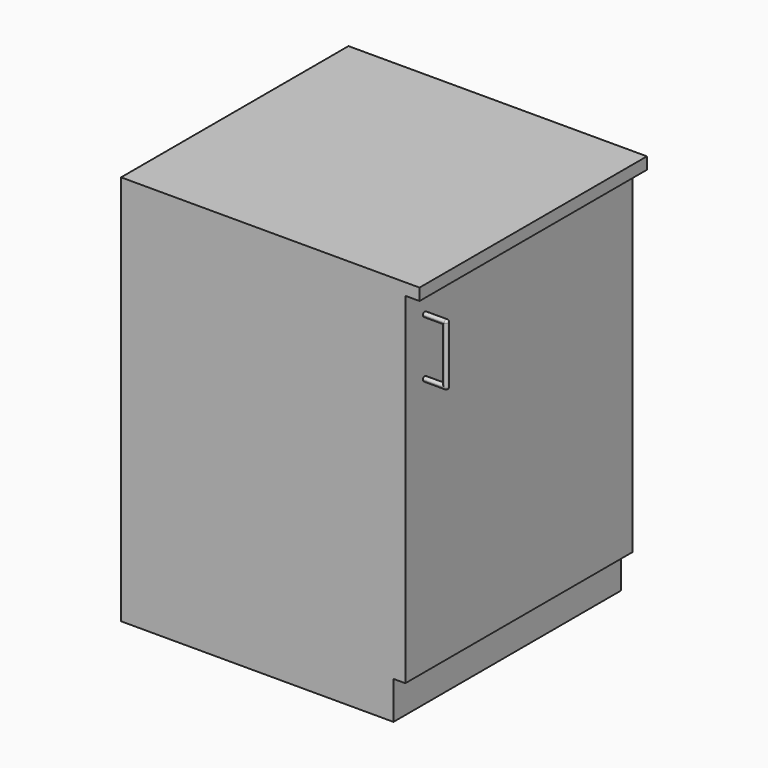
from build123d import *

# Parameters (mm, degrees)
F0_W        = 600
F0_H        = 600
F1_DEPTH    = 800
F2_W        = 600
F2_H        = 80
F3_DEPTH    = 25
F5_DEPTH    = 50
F6_T1_DEPTH = 120
F6_T4_ANGLE = 180
F6_T6_ANGLE = 180
F7_W        = 40
F7_H        = 110
F8_DEPTH    = 25
F9_R        = 4.99999
F10_W       = 630
F10_H       = 600
F11_DEPTH   = 25


# Not quite as in the source:
# - a fillet or chamfer that OpenCascade refuses, or shapes differently, is made with other operations: its cross-section is extruded or revolved along the edge and cut away or added
# - a fillet or chamfer is up to 0.001 mm smaller than in the source, because OpenCascade refuses the exact size


with BuildPart() as f1:
    # F0 (on Top) → F1 (new body)
    with BuildSketch(Plane.XY):
        Rectangle(F0_W, F0_H)
    extrude(amount=F1_DEPTH)

    # F2 (on face) → F3 (cut)
    with BuildSketch(Plane.YZ.offset(300)):
        with Locations((0, 40)):
            Rectangle(F2_W, F2_H)
    extrude(amount=-F3_DEPTH, mode=Mode.SUBTRACT)

    # F4 (on face) → F5 (join)
    with BuildSketch(Plane.YZ.offset(300)):
        with BuildLine():
            ThreePointArc((-248.5795542598, 750), (-252.1150881657, 748.5355339059), (-253.5795542598, 745))
            Line((-253.5795542598, 745), (-253.5795542598, 625))
            ThreePointArc((-253.5795542598, 625), (-252.1150881657, 621.4644660941), (-248.5795542598, 620))
            ThreePointArc((-248.5795542598, 620), (-245.0440203538, 621.4644660941), (-243.5795542598, 625))
            Line((-243.5795542598, 625), (-243.5795542598, 745))
            ThreePointArc((-243.5795542598, 745), (-245.0440203538, 748.5355339059), (-248.5795542598, 750))
        make_face()
    extrude(amount=F5_DEPTH)

    # F6: fillet of radius 5 on 4 edges, made by hand

    # F6_s2 → F6_t1 (cut)
    with BuildSketch(Plane.XY.offset(625)):
        with BuildLine():
            ThreePointArc((345, -253.5795542598), (348.5355339059, -252.1150881657), (350, -248.5795542598))
            Line((350, -248.5795542598), (350, -253.5795542598))
            Line((350, -253.5795542598), (345, -253.5795542598))
        make_face()
        with BuildLine():
            ThreePointArc((345, -243.5795542598), (348.5355339059, -245.0440203538), (350, -248.5795542598))
            Line((350, -248.5795542598), (350, -243.5795542598))
            Line((350, -243.5795542598), (345, -243.5795542598))
        make_face()
    extrude(amount=F6_T1_DEPTH, mode=Mode.SUBTRACT)

    # F6_s3 → F6_t4 (revolve, cut)
    with BuildSketch(Plane.XY.offset(745)):
        with BuildLine():
            ThreePointArc((345, -253.5795542598), (348.5355339059, -252.1150881657), (350, -248.5795542598))
            Line((350, -248.5795542598), (350, -253.5795542598))
            Line((350, -253.5795542598), (345, -253.5795542598))
        make_face()
    revolve(axis=Axis((350, -248.5795542598, 745), (-1, 0, 0)), revolution_arc=F6_T4_ANGLE, mode=Mode.SUBTRACT)

    # F6_s5 → F6_t6 (revolve, cut)
    with BuildSketch(Plane.XY.offset(625)):
        with BuildLine():
            ThreePointArc((345, -243.5795542598), (348.5355339059, -245.0440203538), (350, -248.5795542598))
            Line((350, -248.5795542598), (350, -243.5795542598))
            Line((350, -243.5795542598), (345, -243.5795542598))
        make_face()
    revolve(axis=Axis((350, -248.5795542598, 625), (-1, 0, 0)), revolution_arc=F6_T6_ANGLE, mode=Mode.SUBTRACT)

    # F7 (on face) → F8 (cut)
    with BuildSketch(Plane(origin=(0, -243.5795542598, 0), x_dir=(-1, 0, 0), z_dir=(0, 1, 0))):
        with Locations((-320, 685)):
            Rectangle(F7_W, F7_H)
    extrude(amount=-F8_DEPTH, mode=Mode.SUBTRACT)

    # F9 (radius 5 in the source; OpenCascade refuses exactly that, so slightly less here)
    f9_edges = [f1.edges().sort_by_distance(p)[0] for p in [
        (320, -243.579554, 740),
        (340, -243.579554, 685),
        (320, -243.579554, 630),
        (320, -253.579554, 740),
        (340, -253.579554, 685),
        (320, -253.579554, 630),
    ]]
    fillet(f9_edges, radius=F9_R)

    # F10 (on face) → F11 (join)
    with BuildSketch(Plane.XY.offset(800)):
        with Locations((15, 0)):
            Rectangle(F10_W, F10_H)
    extrude(amount=F11_DEPTH)


solid = f1.part
